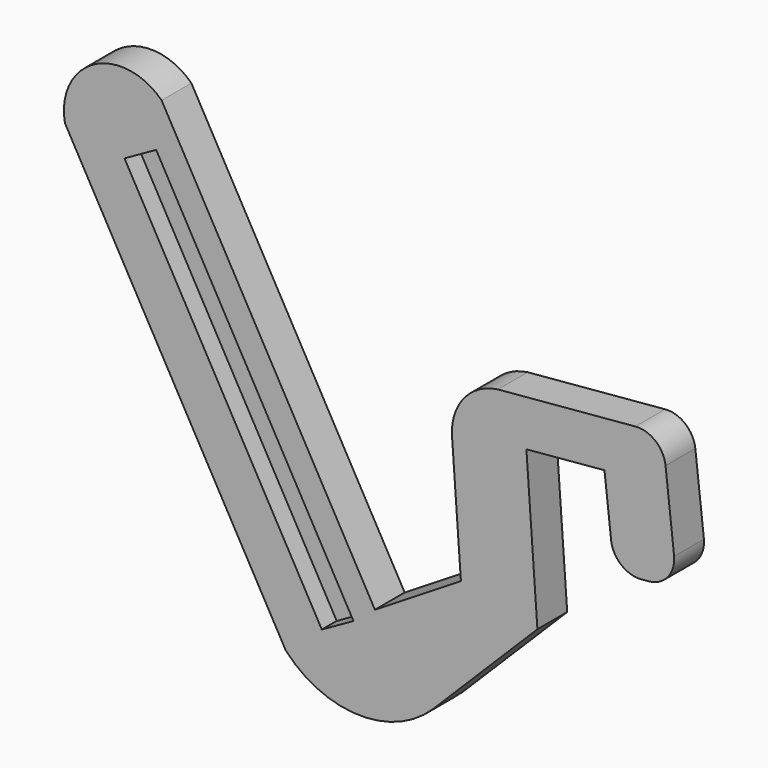
from build123d import *

# Parameters (mm, degrees)
F1_DEPTH = 4
F2_DEPTH = 2


# Not quite as in the source:
# - a feature names something its author has since deleted; it is built from what else it names


with BuildPart() as f1:
    # F0 (on Front) → F1 (new body)
    with BuildSketch(Plane.XZ):
        with BuildLine():
            Line((21.8857619278, 24.0777302796), (22.6911712955, 24.1481944696))
            ThreePointArc((22.6911712955, 24.1481944696), (24.7278373945, 25.2084157357), (25.4182881585, 27.3982457918))
            Line((25.4182881585, 27.3982457918), (24.4967342397, 35.6661240294))
            ThreePointArc((24.4967342397, 35.6661240294), (23.4156220476, 37.6550864329), (21.2523714627, 38.3222610136))
            Line((21.2523714627, 38.3222610136), (6.4843232999, 37.0234552548))
            ThreePointArc((6.4843232999, 37.0234552548), (2.8261843885, 34.9862585866), (1.5612437018, 30.9947581645))
            Line((1.5612437018, 30.9947581645), (2.5138241495, 17.5994470493))
            Line((2.5138241495, 17.5994470493), (-6.7239039322, 11.8946529702))
            Line((-6.7239039322, 11.8946529702), (-29.6357786399, 52.6132809116))
            ThreePointArc((-29.6357786399, 52.6132809116), (-36.8608896735, 53.670290075), (-40.0246161044, 47.0892314299))
            Line((-40.0246161044, 47.0892314299), (-16.300002113, 4.9262158573))
            ThreePointArc((-16.300002113, 4.9262158573), (-8.4430569993, 1.3688058119), (-0.4374276181, 4.5776453154))
            Line((-0.4374276181, 4.5776453154), (10.7330901066, 15.7259296403))
            Line((10.7330901066, 15.7259296403), (9.5491620303, 32.356556315))
            Line((9.5491620303, 32.356556315), (17.93825214, 33.1033145689))
            Line((17.93825214, 33.1033145689), (18.6281962336, 26.9133634004))
            ThreePointArc((18.6281962336, 26.9133634004), (19.654585126, 24.8035187117), (21.8857619278, 24.0777302796))
        make_face()
        Polygon((-9.0293143542, 10.0775616021), (-12.4281861821, 8.1650579296), (-33.6211269399, 45.8288231449), (-30.2222551107, 47.741326818), align=None, mode=Mode.SUBTRACT)
    extrude(amount=F1_DEPTH)

    # F0 (on Front) → F2 (join)
    with BuildSketch(Plane.XZ):
        Polygon((-33.6211269399, 45.8288231449), (-12.4281861821, 8.1650579296), (-9.0293143542, 10.0775616021), (-30.2222551107, 47.741326818), align=None)
    extrude(amount=F2_DEPTH)


solid = f1.part
